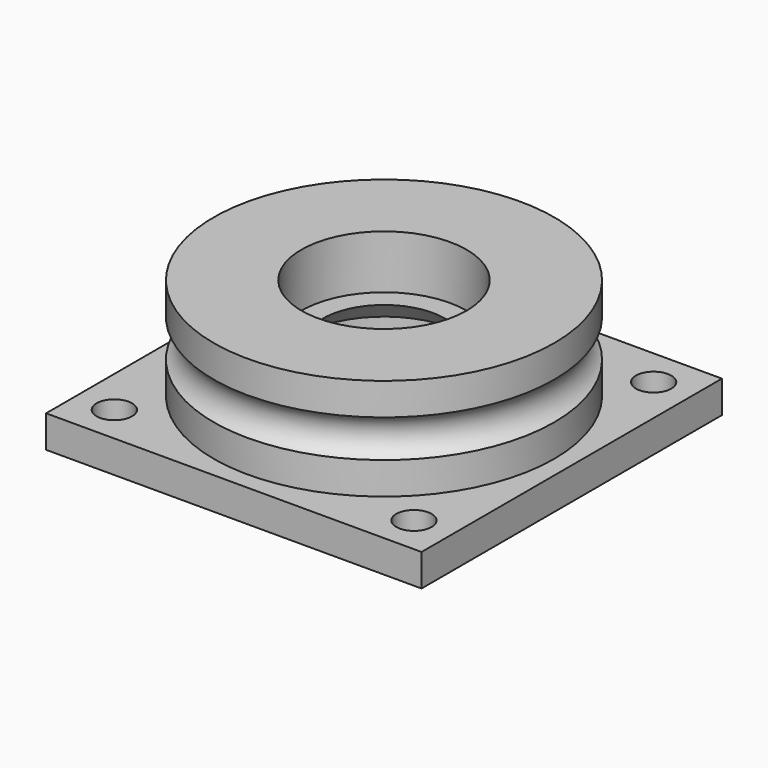
from build123d import *

# Parameters (mm, degrees)
F2_W      = 35
F2_H      = 35
F2_R      = 15.875
F2_R_2    = 7.7
F3_DEPTH  = 3
F4_D      = 3.3
F4_DEPTH  = 13.905
F4_TIP    = 0.9914200214
F5_R      = 15.875
F5_R_2    = 7.7
F6_DEPTH  = 9.5
F10_R     = 7.7
F10_R_2   = 5.7
F11_DEPTH = 2
F12_SIZE  = 1.99999


# Not quite as in the source:
# - a fillet or chamfer is up to 0.001 mm smaller than in the source, because OpenCascade refuses the exact size


with BuildPart() as f3:
    # F2 (on Top) → F3 (new body)
    with BuildSketch(Plane.XY):
        Rectangle(F2_W, F2_H)
        Circle(F2_R, mode=Mode.SUBTRACT)
        Circle(F2_R)
        Circle(F2_R_2, mode=Mode.SUBTRACT)
    extrude(amount=F3_DEPTH)

    # F4
    with Locations(Plane(origin=(0, 0, 0), x_dir=(1, 0, 0), z_dir=(0, 0, -1))):
        with Locations((-13.9644660941, 13.9644660941), (-13.9644660941, -13.9644660941), (13.9644660941, -13.9644660941), (13.9644660941, 13.9644660941)):
            Hole(F4_D / 2, depth=F4_DEPTH)
            with Locations((0, 0, -(F4_DEPTH + F4_TIP / 2))):  # 118° drill point
                Cone(0, F4_D / 2, F4_TIP, mode=Mode.SUBTRACT)

    # F5 (on face) → F6 (join)
    with BuildSketch(Plane.XY.offset(3)):
        Circle(F5_R)
        Circle(F5_R_2, mode=Mode.SUBTRACT)
    extrude(amount=F6_DEPTH)

    # F7 (on Right) → F8 (revolve, cut)
    with BuildSketch(Plane.YZ):
        with BuildLine():
            ThreePointArc((-15.875, 6), (-14.8432458366, 7.75), (-15.875, 9.5))
            Line((-15.875, 9.5), (-15.875, 6))
        make_face()
    revolve(axis=Axis((0, 0, 3), (0, 0, -1)), mode=Mode.SUBTRACT)

    # F10 (on offset) → F11 (join)
    with BuildSketch(Plane.XY.offset(5.5)):
        Circle(F10_R)
        Circle(F10_R_2, mode=Mode.SUBTRACT)
    extrude(amount=F11_DEPTH)

    # F12 (size 2 in the source; OpenCascade refuses exactly that, so slightly less here)
    f12_edges = [f3.edges().sort_by_distance(p)[0] for p in [
        (-5.7, 0, 5.5),
    ]]
    chamfer(f12_edges, length=F12_SIZE)


solid = f3.part
